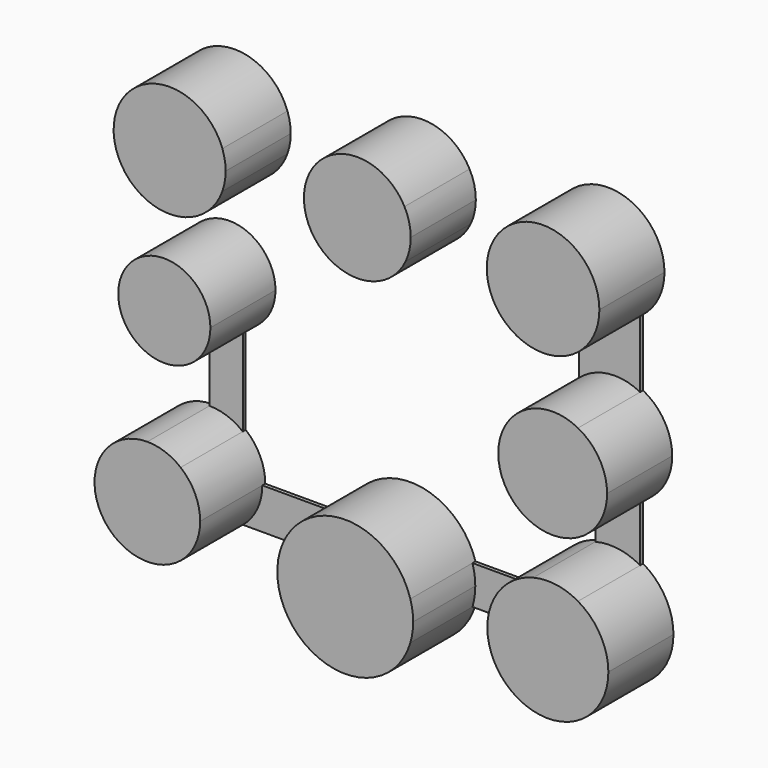
from build123d import *

# Parameters (mm, degrees)
F1_DEPTH = 11
F2_DEPTH = 11
F3_DEPTH = 0.5


# Not quite as in the source:
# - the program builds the solid bodies; features that only make, move or delete a surface that nothing else refers to are left out


with BuildPart() as f1:
    # F0 (on Front) → F1 (new body)
    with BuildSketch(Plane.XZ):
        with BuildLine():
            ThreePointArc((-48.0797858384, 40.2328155244), (-47.7475992787, 41.4908425789), (-47.6357689738, 42.7871735409))
            ThreePointArc((-47.6357689738, 42.7871735409), (-47.7463471065, 44.0762802216), (-48.0748507334, 45.3277229588))
            ThreePointArc((-48.0748507334, 45.3277229588), (-60.375625727, 48.3155165258), (-58.2165755639, 35.8425666648))
            ThreePointArc((-58.2165755639, 35.8425666648), (-55.2660968969, 35.2180036102), (-52.3059486726, 35.7950008925))
            ThreePointArc((-52.3059486726, 35.7950008925), (-49.723681576, 37.5670993069), (-48.0797858384, 40.2328155244))
        make_face()
    extrude(amount=F1_DEPTH)


with BuildPart() as f2:
    # F0 (on Front) → F2 (new body)
    with BuildSketch(Plane.XZ):
        with BuildLine():
            ThreePointArc((-23.456767508, 46.4283592716), (-30.4311757631, 50.2349900835), (-36.6802987427, 45.3277229588))
            ThreePointArc((-36.6802987427, 45.3277229588), (-32.5328439874, 36.3437266645), (-23.3130527419, 39.9366390976))
            ThreePointArc((-23.3130527419, 39.9366390976), (-22.7895849326, 41.4491210345), (-22.612189983, 43.0397659315))
            ThreePointArc((-22.612189983, 43.0397659315), (-22.8265154402, 44.7858956532), (-23.456767508, 46.4283592716))
        make_face()
    extrude(amount=F2_DEPTH)


with BuildPart() as f2b:
    # F0 (on Front) → F2, piece 2 (new body)
    with BuildSketch(Plane.XZ):
        with BuildLine():
            ThreePointArc((0, 36.7466998694), (2.1283855445, 39.4003538773), (2.8884372282, 42.7161080988))
            ThreePointArc((2.8884372282, 42.7161080988), (-8.6637290747, 49.2300143883), (-8.2591603931, 35.9740781474))
            ThreePointArc((-8.2591603931, 35.9740781474), (-4.0151002339, 35.1366227762), (0, 36.7466998694))
        make_face()
    extrude(amount=F2_DEPTH)


with BuildPart() as f2c:
    # F0 (on Front) → F2, piece 3 (new body)
    with BuildSketch(Plane.XZ):
        with BuildLine():
            ThreePointArc((0, 27.7067552004), (-4.2794308504, 28.5019946278), (-8.2591603931, 26.7391313554))
            ThreePointArc((-8.2591603931, 26.7391313554), (-10.6648668946, 19.9029390291), (-6.0418137213, 14.3218702558))
            ThreePointArc((-6.0418137213, 14.3218702558), (-2.9817939053, 13.8533705398), (0, 14.6853070545))
            ThreePointArc((0, 14.6853070545), (2.8730515364, 17.3929499669), (3.9324518182, 21.1960311275))
            ThreePointArc((3.9324518182, 21.1960311275), (2.8730515364, 24.9991122881), (0, 27.7067552004))
        make_face()
    extrude(amount=F2_DEPTH)


with BuildPart() as f2d:
    # F0 (on Front) → F2, piece 4 (new body)
    with BuildSketch(Plane.XZ):
        with BuildLine():
            ThreePointArc((0, 7.0900501454), (-2.9388285364, 8.0987617403), (-6.0418137213, 7.9384645471))
            ThreePointArc((-6.0418137213, 7.9384645471), (-10.5165626716, 5.0401961715), (-12.2543084234, 0))
            ThreePointArc((-12.2543084234, 0), (-11.7698509636, -2.7729589527), (-10.3738746923, -5.2173915319))
            ThreePointArc((-10.3738746923, -5.2173915319), (-1.303128429, -7.6937635819), (4.10213366, 0))
            ThreePointArc((4.10213366, 0), (3.0026993435, 4.0956169141), (0, 7.0900501454))
        make_face()
    extrude(amount=F2_DEPTH)


with BuildPart() as f2e:
    # F0 (on Front) → F2, piece 5 (new body)
    with BuildSketch(Plane.XZ):
        with BuildLine():
            ThreePointArc((-22.2847013796, -2.608695766), (-22.3797796773, -1.2907012663), (-22.6630456746, 0))
            ThreePointArc((-22.6630456746, 0), (-31.4673930407, 6.5739958951), (-40.2717404068, 0))
            ThreePointArc((-40.2717404068, 0), (-40.6484919474, -2.7797191761), (-40.1684777533, -5.5434787162))
            ThreePointArc((-40.1684777533, -5.5434787162), (-31.2963696305, -11.7897946727), (-22.6630456746, -5.2173915319))
            ThreePointArc((-22.6630456746, -5.2173915319), (-22.3797796773, -3.9266902656), (-22.2847013796, -2.608695766))
        make_face()
    extrude(amount=F2_DEPTH)


with BuildPart() as f2f:
    # F0 (on Front) → F2, piece 6 (new body)
    with BuildSketch(Plane.XZ):
        with BuildLine():
            ThreePointArc((-53.7156391117, -5.5434787162), (-51.7695567399, -3.0699403099), (-51.0759463743, 0))
            ThreePointArc((-51.0759463743, 0), (-51.7695567399, 3.0699403099), (-53.7156391117, 5.5434787162))
            ThreePointArc((-53.7156391117, 5.5434787162), (-55.8286204459, 6.7295063399), (-58.2165755639, 7.1406291896))
            ThreePointArc((-58.2165755639, 7.1406291896), (-64.9460819038, -2.387955118), (-53.7156391117, -5.5434787162))
        make_face()
    extrude(amount=F2_DEPTH)


with BuildPart() as f2g:
    # F0 (on Front) → F2, piece 7 (new body)
    with BuildSketch(Plane.XZ):
        with BuildLine():
            ThreePointArc((-58.2165755639, 17.6855820413), (-55.9691628256, 17.2485445266), (-53.7156391117, 17.6528917491))
            ThreePointArc((-53.7156391117, 17.6528917491), (-50.7970881723, 19.9389032943), (-49.6940344894, 23.4782621264))
            ThreePointArc((-49.6940344894, 23.4782621264), (-59.4259467219, 28.6306608138), (-58.2165755639, 17.6855820413))
        make_face()
    extrude(amount=F2_DEPTH)


with BuildPart() as f3:
    # F0 (on Front) → F3 (new body)
    with BuildSketch(Plane.XZ):
        with BuildLine():
            ThreePointArc((-40.1684777533, -5.5434787162), (-40.6484919474, -2.7797191761), (-40.2717404068, 0))
            Line((-40.2717404068, 0), (-51.0759463743, 0))
            ThreePointArc((-51.0759463743, 0), (-51.7695567399, -3.0699403099), (-53.7156391117, -5.5434787162))
            Line((-53.7156391117, -5.5434787162), (-40.1684777533, -5.5434787162))
        make_face()
    extrude(amount=F3_DEPTH)


with BuildPart() as f3b:
    # F0 (on Front) → F3, piece 2 (new body)
    with BuildSketch(Plane.XZ):
        with BuildLine():
            ThreePointArc((-10.3738746923, -5.2173915319), (-11.7698509636, -2.7729589527), (-12.2543084234, 0))
            Line((-12.2543084234, 0), (-22.6630456746, 0))
            ThreePointArc((-22.6630456746, 0), (-22.3797796773, -1.2907012663), (-22.2847013796, -2.608695766))
            ThreePointArc((-22.2847013796, -2.608695766), (-22.3797796773, -3.9266902656), (-22.6630456746, -5.2173915319))
            Line((-22.6630456746, -5.2173915319), (-10.3738746923, -5.2173915319))
        make_face()
    extrude(amount=F3_DEPTH)


with BuildPart() as f3c:
    # F0 (on Front) → F3, piece 3 (new body)
    with BuildSketch(Plane.XZ):
        with BuildLine():
            ThreePointArc((0, 14.6853070545), (-2.9817939053, 13.8533705398), (-6.0418137213, 14.3218702558))
            Line((-6.0418137213, 14.3218702558), (-6.0418137213, 7.9384645471))
            ThreePointArc((-6.0418137213, 7.9384645471), (-2.9388285364, 8.0987617403), (0, 7.0900501454))
            Line((0, 7.0900501454), (0, 14.6853070545))
        make_face()
    extrude(amount=F3_DEPTH)


with BuildPart() as f3d:
    # F0 (on Front) → F3, piece 4 (new body)
    with BuildSketch(Plane.XZ):
        with BuildLine():
            ThreePointArc((0, 36.7466998694), (-4.0151002339, 35.1366227762), (-8.2591603931, 35.9740781474))
            Line((-8.2591603931, 35.9740781474), (-8.2591603931, 26.7391313554))
            ThreePointArc((-8.2591603931, 26.7391313554), (-4.2794308504, 28.5019946278), (0, 27.7067552004))
            Line((0, 27.7067552004), (0, 36.7466998694))
        make_face()
    extrude(amount=F3_DEPTH)


with BuildPart() as f3e:
    # F0 (on Front) → F3, piece 5 (new body)
    with BuildSketch(Plane.XZ):
        with BuildLine():
            ThreePointArc((-58.2165755639, 7.1406291896), (-55.8286204459, 6.7295063399), (-53.7156391117, 5.5434787162))
            Line((-53.7156391117, 5.5434787162), (-53.7156391117, 17.6528917491))
            ThreePointArc((-53.7156391117, 17.6528917491), (-55.9691628256, 17.2485445266), (-58.2165755639, 17.6855820413))
            Line((-58.2165755639, 17.6855820413), (-58.2165755639, 7.1406291896))
        make_face()
    extrude(amount=F3_DEPTH)


solid = Compound([f1.part, f2.part, f2b.part, f2c.part, f2d.part, f2e.part, f2f.part, f2g.part, f3.part, f3b.part, f3c.part, f3d.part, f3e.part])
